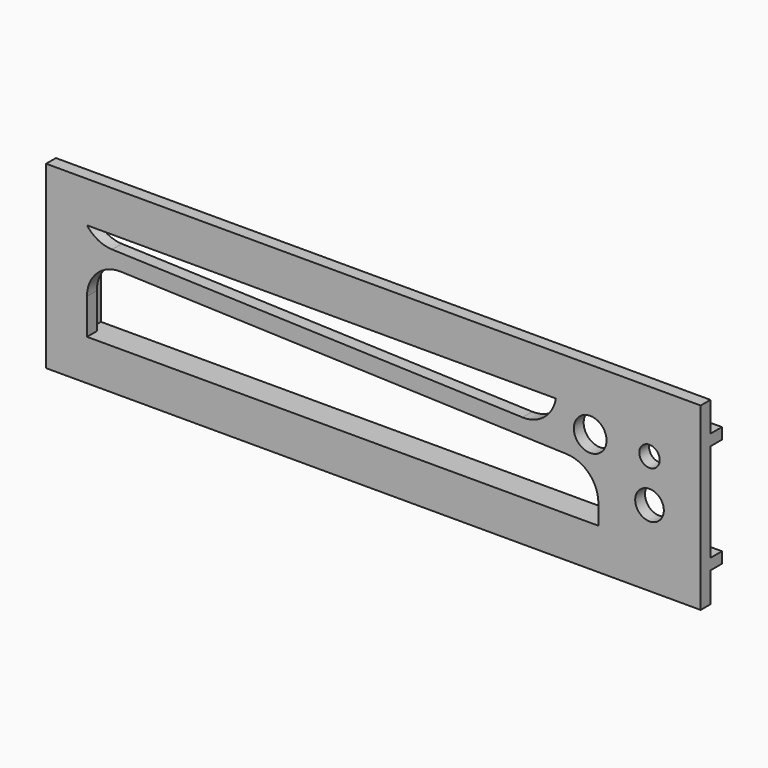
from build123d import *

# Parameters (mm, degrees)
F0_R        = 2.2225
F0_R_2      = 2.54
F0_R_3      = 1.5875
F0_W        = 79.375
F0_H        = 6.35
F1_DEPTH    = 0.9525
F2_T1_DEPTH = 1.905
F3_W        = 3.4798
F3_H        = 1.7145
F3_W_2      = 1.7272
F3_H_2      = 15.24
F3_W_3      = 91.7448
F3_H_3      = 1.7272
F3_W_4      = 2.921
F4_DEPTH    = 3.175


# Not quite as in the source:
# - a fillet or chamfer that OpenCascade refuses, or shapes differently, is made with other operations: its cross-section is extruded or revolved along the edge and cut away or added
# - a feature names something its author has since deleted; it is built from what else it names


with BuildPart() as f1:
    # F0 (on Front) → F1 (new body, symmetric)
    with BuildSketch(Plane.XZ):
        Polygon((-50.8, 27.94), (-50.8, 0), (-44.45, 0), (-44.45, 6.35), (-44.45, 17.145), (34.925, 14.3731639216), (34.925, 6.35), (34.925, 0), (50.8, 0), (50.8, 27.94), align=None)
        with Locations((42.8625, 11.7475)):
            Circle(F0_R, mode=Mode.SUBTRACT)
        Polygon((-44.45, 21.59), (28.3304192035, 21.59), (28.3304192035, 17.145), (-44.45, 19.6865482425), align=None, mode=Mode.SUBTRACT)
        with Locations((33.655, 18.415)):
            Circle(F0_R_2, mode=Mode.SUBTRACT)
        with Locations((42.8625, 18.415)):
            Circle(F0_R_3, mode=Mode.SUBTRACT)
        with Locations((-4.7625, 3.175)):
            Rectangle(F0_W, F0_H)
    extrude(amount=F1_DEPTH, both=True)

    # F2: fillet of radius 5.08 on 4 edges, made by hand

    # F2_s2 → F2_t1 (join)
    with BuildSketch(Plane.XZ.offset(-0.9525)):
        with BuildLine():
            ThreePointArc((-39.1927105568, 16.9614114072), (-42.8988645219, 15.5387521917), (-44.45, 11.8845060059))
            Line((-44.45, 11.8845060059), (-44.45, 17.145))
            Line((-44.45, 17.145), (-39.1927105568, 16.9614114072))
        make_face()
        with BuildLine():
            ThreePointArc((34.925, 9.4674649456), (33.4992461857, 12.9963294675), (30.0222894432, 14.5443703468))
            Line((30.0222894432, 14.5443703468), (34.925, 14.3731639216))
            Line((34.925, 14.3731639216), (34.925, 9.4674649456))
        make_face()
        with BuildLine():
            ThreePointArc((-44.45, 21.59), (-42.7347440797, 20.1271540197), (-40.5553991831, 19.5505457851))
            Line((-40.5553991831, 19.5505457851), (-44.45, 19.6865482425))
            Line((-44.45, 19.6865482425), (-44.45, 21.59))
        make_face()
        with BuildLine():
            ThreePointArc((28.3304192035, 21.59), (26.5399663684, 18.4773950775), (23.1386411982, 17.326300883))
            Line((23.1386411982, 17.326300883), (28.3304192035, 17.145))
            Line((28.3304192035, 17.145), (28.3304192035, 21.59))
        make_face()
    extrude(amount=F2_T1_DEPTH)

    # F3 (on Front) → F4 (join)
    with BuildSketch(Plane.XZ):
        with Locations((-49.0601, 5.49275)):
            Rectangle(F3_W, F3_H)
        with Locations((-46.4566, 13.97)):
            Rectangle(F3_W_2, F3_H_2)
        with Locations((-46.4566, 5.49275)):
            Rectangle(F3_W_2, F3_H)
        with Locations((0.2794, 5.49275)):
            Rectangle(F3_W_3, F3_H)
        with Locations((-46.4566, 22.4536)):
            Rectangle(F3_W_2, F3_H_3)
        with Locations((-49.0601, 22.4536)):
            Rectangle(F3_W, F3_H_3)
        with Locations((47.0154, 13.97)):
            Rectangle(F3_W_2, F3_H_2)
        with Locations((47.0154, 5.49275)):
            Rectangle(F3_W_2, F3_H)
        with Locations((0.2794, 22.4536)):
            Rectangle(F3_W_3, F3_H_3)
        with Locations((49.3395, 5.49275)):
            Rectangle(F3_W_4, F3_H)
        with Locations((47.0154, 22.4536)):
            Rectangle(F3_W_2, F3_H_3)
        with Locations((49.3395, 22.4536)):
            Rectangle(F3_W_4, F3_H_3)
    extrude(amount=-F4_DEPTH)


solid = f1.part
